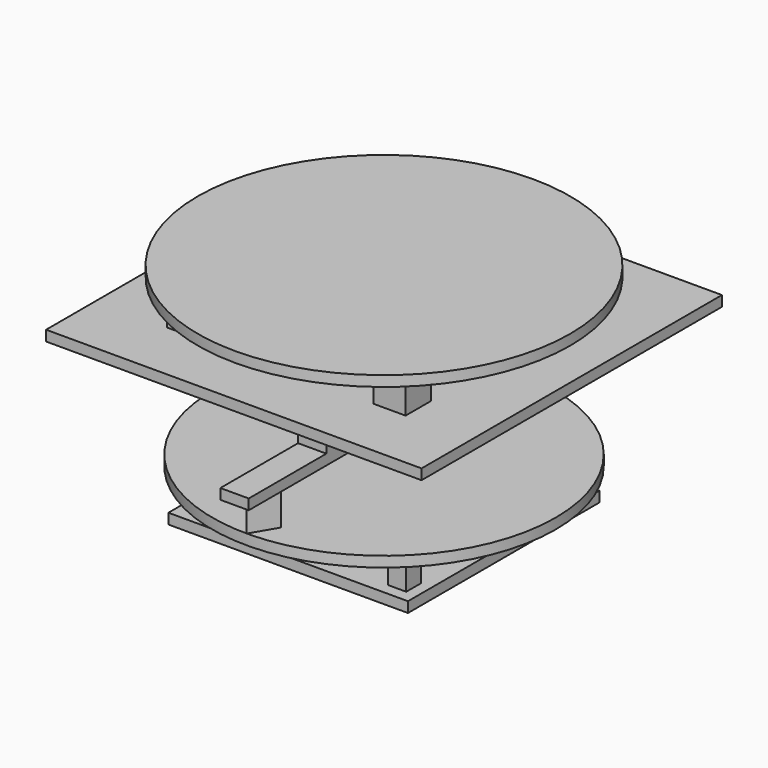
from build123d import *

# Parameters (mm, degrees)
F0_W      = 58.42
F0_H      = 58.42
F1_DEPTH  = 2.54
F2_W      = 4.4949427247
F2_H      = 4.4949445873
F3_DEPTH  = 7.62
F4_W      = 4.4949445873
F4_H      = 4.4949445873
F5_DEPTH  = 7.62
F6_W      = 4.4949427247
F6_H      = 4.49494645
F7_DEPTH  = 7.62
F8_W      = 4.4949445873
F8_H      = 4.49494645
F9_DEPTH  = 7.62
F10_R     = 41.8491374304
F11_DEPTH = 2.54
F13_DEPTH = 7.62
F15_DEPTH = 7.62
F16_W     = 6.9088
F16_H     = 91.0975262523
F17_DEPTH = 2.54
F18_W     = 6.9088
F18_H     = 6.8922471255
F19_DEPTH = 7.62
F20_W     = 6.9088
F20_H     = 6.8922471255
F21_DEPTH = 7.62
F22_W     = 58.42
F22_H     = 58.42
F23_DEPTH = 2.54
F24_R     = 3.8886710073
F24_R_2   = 3.8886723427
F24_R_3   = 3.8886735446
F24_R_4   = 4.0259
F25_DEPTH = 7.62
F26_W     = 91.567
F26_H     = 91.567
F27_DEPTH = 2.54
F28_W     = 7.791236043
F28_H     = 7.791236043
F28_W_2   = 7.7912285924
F28_W_3   = 7.7912434936
F28_H_2   = 7.7912397683
F29_DEPTH = 7.62
F30_R     = 45.4175170009
F31_DEPTH = 2.54


with BuildPart() as f1:
    # F0 (on Top) → F1 (new body)
    with BuildSketch(Plane.XY):
        Rectangle(F0_W, F0_H)
    extrude(amount=F1_DEPTH)

    # F2 (on face) → F3 (join)
    with BuildSketch(Plane.XY.offset(2.54)):
        with Locations((-24.572359398, 24.7221915051)):
            Rectangle(F2_W, F2_H)
    extrude(amount=F3_DEPTH)

    # F4 (on face) → F5 (join)
    with BuildSketch(Plane.XY.offset(2.54)):
        with Locations((24.2726961151, 24.7221915051)):
            Rectangle(F4_W, F4_H)
    extrude(amount=F5_DEPTH)

    # F6 (on face) → F7 (join)
    with BuildSketch(Plane.XY.offset(2.54)):
        with Locations((-24.572359398, -24.1228658706)):
            Rectangle(F6_W, F6_H)
    extrude(amount=F7_DEPTH)

    # F8 (on face) → F9 (join)
    with BuildSketch(Plane.XY.offset(2.54)):
        with Locations((24.2726961151, -24.1228658706)):
            Rectangle(F8_W, F8_H)
    extrude(amount=F9_DEPTH)

    # F10 (on face) → F11 (join)
    with BuildSketch(Plane.XY.offset(10.16)):
        Circle(F10_R)
    extrude(amount=F11_DEPTH)


with BuildPart() as f13:
    # F12 (on face) → F13 (new body)
    with BuildSketch(Plane.XY.offset(12.7)):
        Polygon((3.445815184, 35.8709057852), (0, 41.8491374304), (-3.462984816, 35.8709057852), align=None)
    extrude(amount=F13_DEPTH)



with BuildPart() as f15:
    # F14 (on face) → F15 (new body)
    with BuildSketch(Plane.XY.offset(12.7)):
        Polygon((-3.3829984536, -35.8252816135), (0, -41.8491374304), (3.5258015464, -35.8252816135), align=None)
    extrude(amount=F15_DEPTH)


with BuildPart() as f13_1:
    add(f13.part)

    add(f15.part)  # F17 merges F15
    # F16 (on face) → F17 (join)
    with BuildSketch(Plane.XY.offset(20.32)):
        with Locations((-0.008584816, 0)):
            Rectangle(F16_W, F16_H)
    extrude(amount=F17_DEPTH)

    # F18 (on face) → F19 (join)
    with BuildSketch(Plane.XY.offset(22.86)):
        with Locations((-0.008584816, 19.0285956487)):
            Rectangle(F18_W, F18_H)
    extrude(amount=F19_DEPTH)

    # F20 (on face) → F21 (join)
    with BuildSketch(Plane.XY.offset(22.86)):
        with Locations((-0.008584816, -18.4292690828)):
            Rectangle(F20_W, F20_H)
    extrude(amount=F21_DEPTH)

    # F22 (on face) → F23 (join)
    with BuildSketch(Plane.XY.offset(30.48)):
        Rectangle(F22_W, F22_H)
    extrude(amount=F23_DEPTH)

    # F24 (on face) → F25 (join)
    with BuildSketch(Plane.XY.offset(33.02)):
        with Locations((-22.114558397, 22.2694298633)):
            Circle(F24_R)
        with Locations((-22.114558397, -21.665063095)):
            Circle(F24_R_2)
        with Locations((21.8199381546, -21.665063095)):
            Circle(F24_R_3)
        with Locations((21.8199381546, 22.2694298633)):
            Circle(F24_R_4)
    extrude(amount=F25_DEPTH)

    # F26 (on face) → F27 (join)
    with BuildSketch(Plane.XY.offset(40.64)):
        Rectangle(F26_W, F26_H)
    extrude(amount=F27_DEPTH)

    # F28 (on face) → F29 (join)
    with BuildSketch(Plane.XY.offset(43.18)):
        with Locations((-24.4225282222, 26.2462347746)):
            Rectangle(F28_W, F28_H)
        with Locations((25.9208455682, 26.2462347746)):
            Rectangle(F28_W_2, F28_H)
        with Locations((25.9208455682, -26.7941039056)):
            Rectangle(F28_W_3, F28_H)
        with Locations((-24.4225282222, -26.7941039056)):
            Rectangle(F28_W, F28_H_2)
    extrude(amount=F29_DEPTH)

    # F30 (on face) → F31 (join)
    with BuildSketch(Plane.XY.offset(50.8)):
        Circle(F30_R)
    extrude(amount=F31_DEPTH)


solid = Compound([f1.part, f13_1.part])
